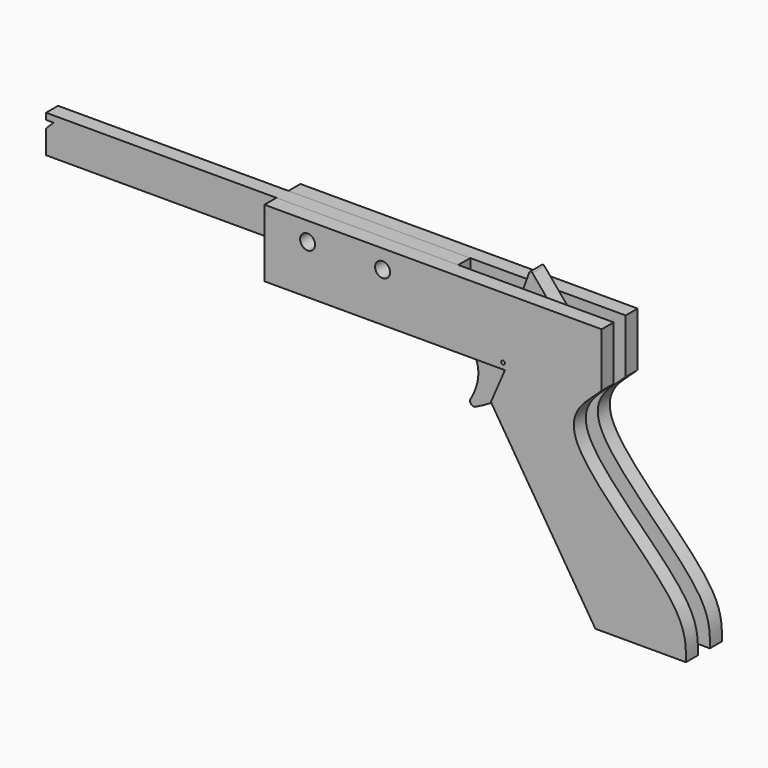
from build123d import *

# Parameters (mm, degrees)
F0_R      = 2.54
F1_DEPTH  = 2.54
F2_W      = 61.6293519594
F2_H      = 12.7
F2_R      = 2.54
F3_DEPTH  = 5.08
F4_R      = 0.635
F5_DEPTH  = 2.54
F6_DEPTH  = 7.6210001
F8_R      = 1.27
F9_R      = 1.27
F10_DEPTH = 2.54
F11_R     = 0.635


# Not quite as in the source:
# - the program builds the solid bodies; features that only make, move or delete a surface that nothing else refers to are left out


with BuildPart() as f1:
    # F0 (on Front) → F1 (new body, symmetric)
    with BuildSketch(Plane.XZ):
        Polygon((-139.7, 0), (0, 0), (0, 12.7), (-139.7, 12.7), (-139.7, 10.5376646731), (-137.1728569348, 10.5376646731), (-139.7, 8.0105216078), align=None)
        with Locations((-46.99, 6.35)):
            Circle(F0_R, mode=Mode.SUBTRACT)
        with Locations((-21.59, 6.35)):
            Circle(F0_R, mode=Mode.SUBTRACT)
    extrude(amount=F1_DEPTH, both=True)


with BuildPart() as f3:
    # F2 (on face) → F3 (new body)
    with BuildSketch(Plane.XZ.offset(2.54)):
        with BuildLine():
            Line((52.6706480406, 12.7), (0, 12.7))
            Line((0, 12.7), (0, 0))
            Line((0, 0), (-61.6293519594, 0))
            Line((-61.6293519594, 0), (-61.6293519594, -10.16))
            Line((-61.6293519594, -10.16), (19.8817028996, -10.16))
            Line((19.8817028996, -10.16), (15.1211905229, -21.1940087392))
            Line((15.1211905229, -21.1940087392), (50.5158929033, -77.355248563))
            Line((50.5158929033, -77.355248563), (81.2204327985, -77.355248563))
            add(Edge.make_bspline(
                [(47.799121146, -10.16), (44.3482648072, -13.3692479995), (37.1454276866, -25.357169668), (81.4992006887, -59.9064139099), (81.2842977033, -72.8161541739), (81.2204327985, -77.355248563)],
                knots=[0, 0, 0, 0, 0.2471584038, 0.7295165006, 1, 1, 1, 1], degree=3))
            Line((47.799121146, -10.16), (52.6706480406, -5.6295483074))
            Line((52.6706480406, -5.6295483074), (52.6706480406, 12.7))
        make_face()
        with Locations((-30.8146759797, 6.35)):
            Rectangle(F2_W, F2_H)
        with Locations((-46.99, 6.35)):
            Circle(F2_R, mode=Mode.SUBTRACT)
        with Locations((-21.59, 6.35)):
            Circle(F2_R, mode=Mode.SUBTRACT)
    extrude(amount=F3_DEPTH)

    # F4 (on Front) → F6 (cut, through all)
    with BuildSketch(Plane.XZ):
        with Locations((19.2364566028, -8.0991536379)):
            Circle(F4_R)
    extrude(amount=F6_DEPTH, mode=Mode.SUBTRACT)


with BuildPart() as f5:
    # F4 (on Front) → F5 (new body, symmetric)
    with BuildSketch(Plane.XZ):
        with BuildLine():
            add(Edge.make_bspline(
                [(22.8122286499, -3.9173178375), (19.2917461197, -21.5543570618), (13.5305089255, -24.243020763), (1.8707671043, -29.552931826)],
                knots=[0, 0, 0, 0, 33.1018053319, 33.1018053319, 33.1018053319, 33.1018053319], degree=3))
            Line((22.8122286499, -3.9173178375), (2.2755871012, -8.3797141855))
            add(Edge.make_bspline(
                [(2.2755871012, -8.3797141855), (10.3401988745, -15.254676342), (5.9748672721, -23.7269168006), (1.8707671043, -29.552931826)],
                knots=[0, 0, 0, 0, 21.1770872521, 21.1770872521, 21.1770872521, 21.1770872521], degree=3))
        make_face()
        with Locations((19.2364566028, -8.0991536379)):
            Circle(F4_R, mode=Mode.SUBTRACT)
    extrude(amount=F5_DEPTH, both=True)

    # F8
    f8_edges = [f5.edges().sort_by_distance(p)[0] for p in [
        (1.870767, 1.27, -29.552932),
        (1.870767, -1.27, -29.552932),
    ]]
    fillet(f8_edges, radius=F8_R)


with BuildPart() as f7_1:
    # F7: instance of F3
    add(f3.part.mirror(Plane.XZ))


with BuildPart() as f10:
    # F9 (on Front) → F10 (new body, symmetric)
    with BuildSketch(Plane.XZ):
        Polygon((18.4256873853, 2.853382407), (35.6970995837, 5.8810384254), (24.4393664586, 19.3246921392), align=None)
        with Locations((26.1873844759, 9.3530376572)):
            Circle(F9_R, mode=Mode.SUBTRACT)
    extrude(amount=F10_DEPTH, both=True)

    # F11
    f11_edges = [f10.edges().sort_by_distance(p)[0] for p in [
        (24.439366, 0, 19.324692),
        (35.6971, 0, 5.881038),
        (18.425687, 0, 2.853382),
    ]]
    fillet(f11_edges, radius=F11_R)


solid = Compound([f1.part, f3.part, f5.part, f7_1.part, f10.part])
